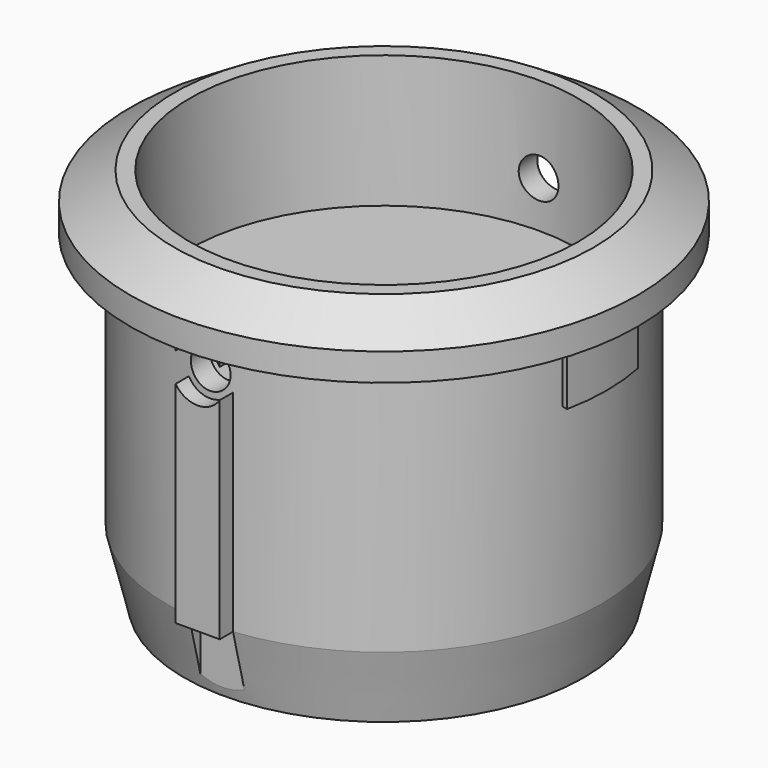
from build123d import *

# Parameters (mm, degrees)
F0_R           = 11.5
F1_DEPTH       = 2.5
F2_R           = 9.85
F3_DEPTH       = 14.8
F4_SIZE2       = 3.2
F4_SIZE        = 0.8
F5_SIZE2       = 1.25
F5_SIZE        = 2
F6_R           = 8.8
F7_DEPTH       = 6
F8_W           = 0.8
F8_H           = 5
F9_DEPTH       = 5
F11_DEPTH      = 11.6
F12_W          = 2
F12_H          = 1.4
F13_DEPTH      = 3.2
F14_R          = 0.9
F15_DEPTH      = 22.0501071022
F17_END_RADIUS = 9.85
F16_R          = 1.2
F17_REACH      = 25.4442196519
F19_DEPTH      = 3


with BuildPart() as f1:
    # F0 (on Top) → F1 (new body)
    with BuildSketch(Plane.XY):
        Circle(F0_R)
    extrude(amount=F1_DEPTH)

    # F2 (on face) → F3 (join)
    with BuildSketch(Plane(origin=(0, 0, 0), x_dir=(1, 0, 0), z_dir=(0, 0, -1))):
        Circle(F2_R)
    extrude(amount=F3_DEPTH)

    # F4
    f4_edges = [f1.edges().sort_by_distance(p)[0] for p in [
        (-9.85, 0, -14.8),
    ]]
    f4_side = f1.faces().sort_by_distance((0, 0, -14.8))[0]
    chamfer(f4_edges, length=F4_SIZE, length2=F4_SIZE2, reference=f4_side)

    # F5
    f5_edges = [f1.edges().sort_by_distance(p)[0] for p in [
        (-11.5, 0, 2.5),
    ]]
    f5_side = f1.faces().sort_by_distance((0, 0, 2.5))[0]
    chamfer(f5_edges, length=F5_SIZE, length2=F5_SIZE2, reference=f5_side)

    # F6 (on face) → F7 (cut)
    with BuildSketch(Plane.XY.offset(2.5)):
        Circle(F6_R)
    extrude(amount=-F7_DEPTH, mode=Mode.SUBTRACT)

    # F8 (on face) → F9 (cut)
    with BuildSketch(Plane(origin=(0, 0, -14.8), x_dir=(1, 0, 0), z_dir=(0, 0, -1))):
        with Locations((-7.1, 0)):
            Rectangle(F8_W, F8_H)
        Rectangle(F8_W, F8_H)
        with Locations((7.1, 0)):
            Rectangle(F8_W, F8_H)
    extrude(amount=-F9_DEPTH, mode=Mode.SUBTRACT)

    # F10 (on face) → F11 (join)
    with BuildSketch(Plane(origin=(0, 0, 0), x_dir=(1, 0, 0), z_dir=(0, 0, -1))):
        with BuildLine():
            Line((-1, 10.5491071022), (-1, 9.7991071022))
            ThreePointArc((-1, 9.7991071022), (0, 9.85), (1, 9.7991071022))
            Line((1, 9.7991071022), (1, 10.5491071022))
            Line((1, 10.5491071022), (-1, 10.5491071022))
        make_face()
    extrude(amount=F11_DEPTH)

    # F12 (on face) → F13 (cut, through all)
    with BuildSketch(Plane(origin=(0, 0, -14.8), x_dir=(1, 0, 0), z_dir=(0, 0, -1))):
        with Locations((0, 9.8491071022)):
            Rectangle(F12_W, F12_H)
    extrude(amount=-F13_DEPTH, mode=Mode.SUBTRACT)

    # F14 (on face) → F15 (cut, through all)
    with BuildSketch(Plane.XZ.offset(10.5491071022)):
        with Locations((0, -1.4)):
            Circle(F14_R)
    extrude(amount=-F15_DEPTH, mode=Mode.SUBTRACT)

    f17_end = (Plane.XY.offset(-5.8) * Cylinder(F17_END_RADIUS, 124.5712732194, mode=Mode.PRIVATE)).faces().sort_by_distance((0, 9.85, -5.8))[0]
    # F16 (on face) → F17 (cut, up to the whole of a round face its end follows)
    with BuildSketch(Plane.XZ.offset(10.5491071022)):
        with Locations((0, -1.4)):
            Circle(F16_R)
    f17_long = extrude(amount=-F17_REACH, mode=Mode.PRIVATE)
    add(split(f17_long, bisect_by=f17_end, keep=Keep.ALL, mode=Mode.PRIVATE).solids().sort_by_distance((0, -10.5491071022, -1.4))[0], mode=Mode.SUBTRACT)

    # F18 (on face) → F19 (join)
    with BuildSketch(Plane(origin=(0, 0, 0), x_dir=(1, 0, 0), z_dir=(0, 0, -1))):
        with BuildLine():
            Line((-9.654950495, 1.9504950495), (-9.9, 2))
            ThreePointArc((-9.9, 2), (-10.1, 0), (-9.9, -2))
            Line((-9.9, -2), (-9.654950495, -1.9504950495))
            ThreePointArc((-9.654950495, -1.9504950495), (-9.85, 0), (-9.654950495, 1.9504950495))
        make_face()
        with BuildLine():
            Line((9.654950495, -1.9504950495), (9.9, -2))
            ThreePointArc((9.9, -2), (10.1, 0), (9.9, 2))
            Line((9.9, 2), (9.654950495, 1.9504950495))
            ThreePointArc((9.654950495, 1.9504950495), (9.85, 0), (9.654950495, -1.9504950495))
        make_face()
    extrude(amount=F19_DEPTH)


solid = f1.part
